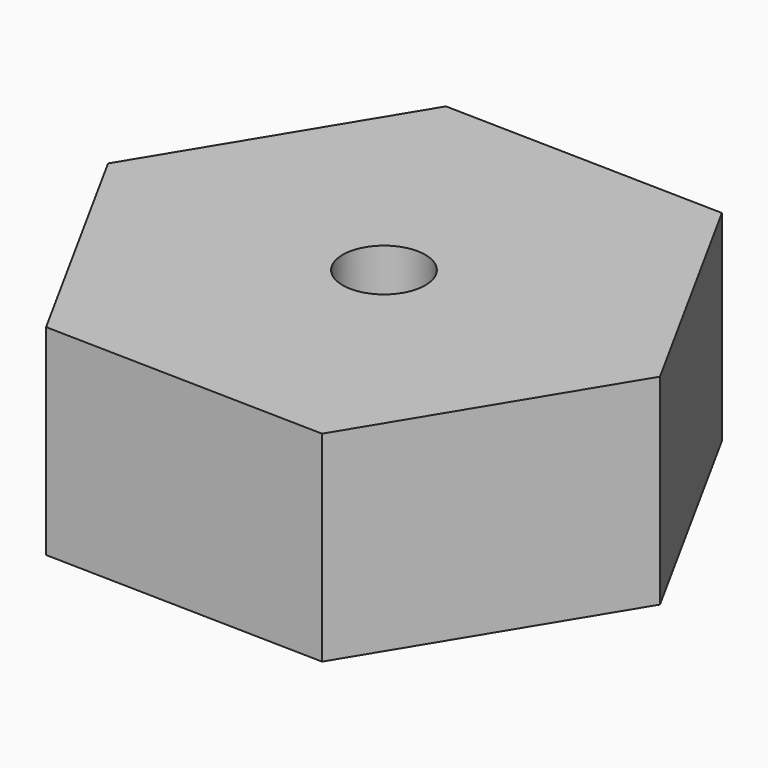
from build123d import *

# Parameters (mm, degrees)
F1_DEPTH = 25
F3_D     = 10.3
F3_DEPTH = 35.25
F3_TIP   = 3.094432188


with BuildPart() as f1:
    # F0 (on Top) → F1 (new body)
    with BuildSketch(Plane.XY):
        Polygon((-16.8322891958, 30.6867078786), (-34.9916131793, 0.7661638919), (-18.1593239835, -29.9205439867), (16.8322891958, -30.6867078786), (34.9916131793, -0.7661638919), (18.1593239835, 29.9205439867), align=None)
    extrude(amount=F1_DEPTH)

    # F3
    with Locations(Plane(origin=(0, 0, 0), x_dir=(1, 0, 0), z_dir=(0, 0, -1))):
        with Locations((0, 0)):
            Hole(F3_D / 2, depth=F3_DEPTH)
            with Locations((0, 0, -(F3_DEPTH + F3_TIP / 2))):  # 118° drill point
                Cone(0, F3_D / 2, F3_TIP, mode=Mode.SUBTRACT)


solid = f1.part
